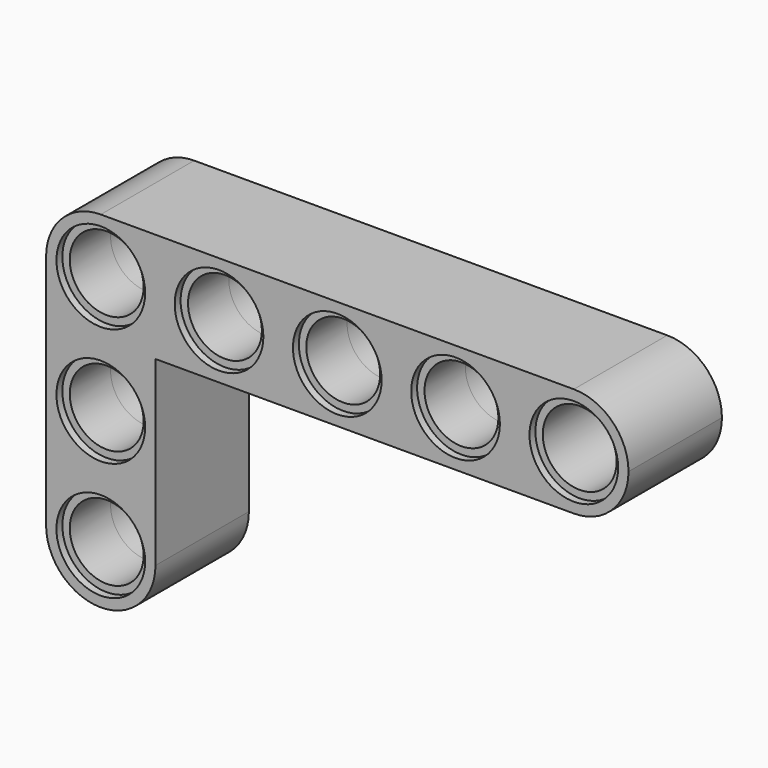
from build123d import *

# Parameters (mm, degrees)
F0_R     = 3
F1_DEPTH = 3.95
F0_R_2   = 2.499
F2_DEPTH = 3.45
F3_R     = 3.69999
F4_R     = 3
F4_W     = 7.4
F4_H     = 7.4
F5_DEPTH = 7.9
F7_R     = 3.69999
F8_R     = 3.7


# Not quite as in the source:
# - a fillet or chamfer is up to 0.001 mm smaller than in the source, because OpenCascade refuses the exact size


with BuildPart() as f1:
    # F0 (on Front) → F1 (new body, symmetric)
    with BuildSketch(Plane.XZ):
        Polygon((19.7, -3.7), (19.7, 3.7), (-19.7, 3.7), (-19.7, -3.7), (-19.7, -19.7), (-12.3, -19.7), (-12.3, -3.7), align=None)
        with Locations((-16, -16)):
            Circle(F0_R, mode=Mode.SUBTRACT)
        with Locations((-16, -8)):
            Circle(F0_R, mode=Mode.SUBTRACT)
        with Locations((-16, 0)):
            Circle(F0_R, mode=Mode.SUBTRACT)
        with Locations((-8, 0)):
            Circle(F0_R, mode=Mode.SUBTRACT)
        Circle(F0_R, mode=Mode.SUBTRACT)
        with Locations((8, 0)):
            Circle(F0_R, mode=Mode.SUBTRACT)
        with Locations((16, 0)):
            Circle(F0_R, mode=Mode.SUBTRACT)
    extrude(amount=F1_DEPTH, both=True)

    # F0 (on Front) → F2 (join, symmetric)
    with BuildSketch(Plane.XZ):
        with Locations((-16, -16)):
            Circle(F0_R)
        with Locations((-16, -16)):
            Circle(F0_R_2, mode=Mode.SUBTRACT)
        with Locations((-16, -8)):
            Circle(F0_R)
        with Locations((-16, -8)):
            Circle(F0_R_2, mode=Mode.SUBTRACT)
        with Locations((-16, 0)):
            Circle(F0_R)
        with Locations((-16, 0)):
            Circle(F0_R_2, mode=Mode.SUBTRACT)
        with Locations((-8, 0)):
            Circle(F0_R)
        with Locations((-8, 0)):
            Circle(F0_R_2, mode=Mode.SUBTRACT)
        Circle(F0_R)
        Circle(F0_R_2, mode=Mode.SUBTRACT)
        with Locations((8, 0)):
            Circle(F0_R)
        with Locations((8, 0)):
            Circle(F0_R_2, mode=Mode.SUBTRACT)
        with Locations((16, 0)):
            Circle(F0_R)
        with Locations((16, 0)):
            Circle(F0_R_2, mode=Mode.SUBTRACT)
    extrude(amount=F2_DEPTH, both=True)

    # F3 (radius 3.7 in the source; OpenCascade refuses exactly that, so slightly less here)
    f3_edges = [f1.edges().sort_by_distance(p)[0] for p in [
        (19.7, 0, 3.7),
        (19.7, 0, -3.7),
    ]]
    fillet(f3_edges, radius=F3_R)

    # F7 (radius 3.7 in the source; OpenCascade refuses exactly that, so slightly less here)
    f7_edges = [f1.edges().sort_by_distance(p)[0] for p in [
        (-12.3, 0, -19.7),
        (-19.7, 0, -19.7),
    ]]
    fillet(f7_edges, radius=F7_R)

    # F8
    f8_edges = [f1.edges().sort_by_distance(p)[0] for p in [
        (-19.7, 0, 3.7),
    ]]
    fillet(f8_edges, radius=F8_R)


with BuildPart() as f5:
    # F4 (on face) → F5 (new body)
    with BuildSketch(Plane.XZ.offset(3.95)):
        Polygon((-12.3, -19.7), (-12.3, -3.7), (-19.7, -3.7), (-19.7, -12.3), (-19.7, -19.7), align=None)
        with Locations((-16, -16)):
            Circle(F4_R, mode=Mode.SUBTRACT)
        with Locations((-16, -8)):
            Circle(F4_R, mode=Mode.SUBTRACT)
        with Locations((-23.4, -16)):
            Rectangle(F4_W, F4_H)
    extrude(amount=F5_DEPTH)


solid = f1.part
